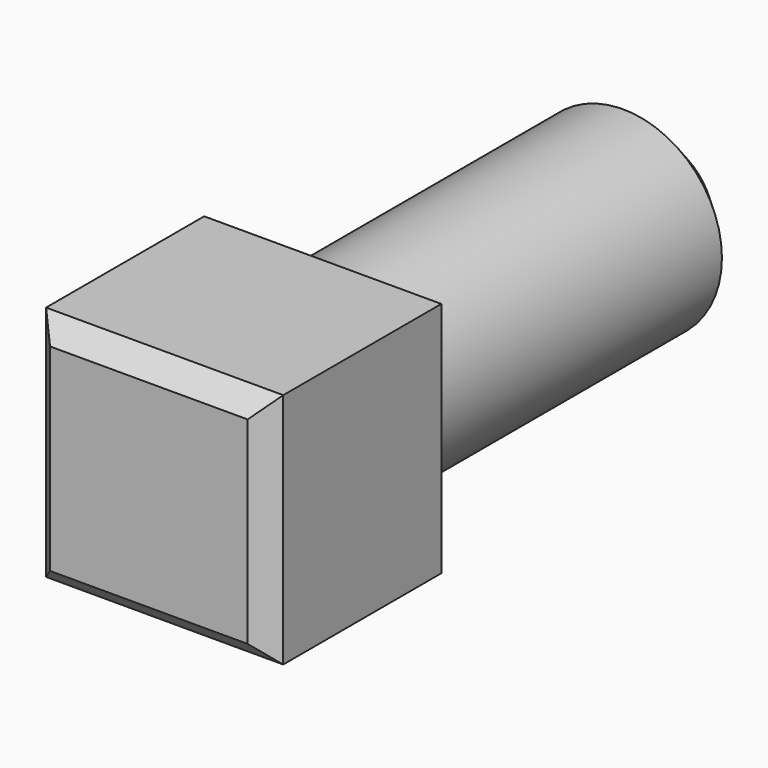
from build123d import *

# Parameters (mm, degrees)
F0_R          = 2.5
F1_DEPTH      = 10
F1_DEPTH_BACK = 6
F2_SIZE       = 1
F0_W          = 6
F0_H          = 6
F3_DEPTH      = 6
F4_SIZE       = 0.49999


# Not quite as in the source:
# - a fillet or chamfer is up to 0.001 mm smaller than in the source, because OpenCascade refuses the exact size


with BuildPart() as f1:
    # F0 (on Front) → F1 (new body, two sides)
    with BuildSketch(Plane.XZ) as f1_sk:
        Circle(F0_R)
    extrude(amount=-F1_DEPTH)
    extrude(f1_sk.sketch, amount=F1_DEPTH_BACK)

    # F2
    f2_edges = [f1.edges().sort_by_distance(p)[0] for p in [
        (-2.5, 10, 0),
    ]]
    chamfer(f2_edges, length=F2_SIZE)

    # F0 (on Front) → F3 (join)
    with BuildSketch(Plane.XZ):
        Rectangle(F0_W, F0_H)
        Circle(F0_R, mode=Mode.SUBTRACT)
    extrude(amount=F3_DEPTH)

    # F4 (size 0.5 in the source; OpenCascade refuses exactly that, so slightly less here)
    f4_edges = [f1.edges().sort_by_distance(p)[0] for p in [
        (3, -6, 0),
        (0, -6, 3),
        (-3, -6, 0),
        (0, -6, -3),
        (3, 0, 0),
        (-3, 0, 0),
        (0, 0, 3),
        (0, 0, -3),
    ]]
    chamfer(f4_edges, length=F4_SIZE)


solid = f1.part
